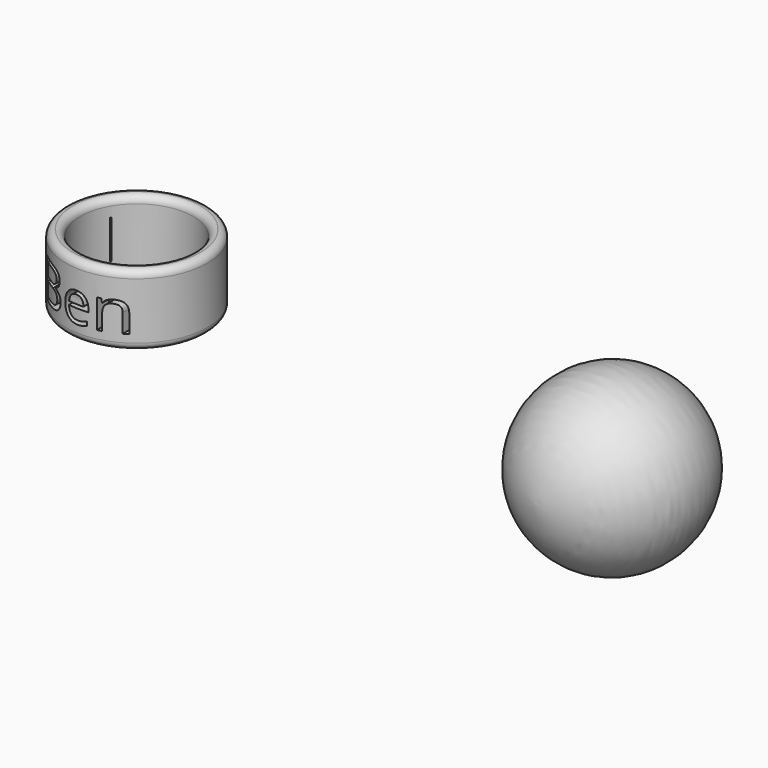
from build123d import *

# Parameters (mm, degrees)
F0_R         = 12.7
F0_R_2       = 10.1142841189
F1_DEPTH     = 12.7
F2_R         = 1.27
F3_TEXT_SIZE = 9.663044087
F4_DEPTH     = 25.4


# Not quite as in the source:
# - Text() gives the source's letters only with a copy of the font that has no kerning and outlines rounded to 1/6400 em; it was checked with that copy


with BuildPart() as f1:
    # F0 (on Top) → F1 (new body)
    with BuildSketch(Plane.XY):
        with Locations((-45.8856523037, 20.2095657587)):
            Circle(F0_R)
        with Locations((-45.8856523037, 20.2095657587)):
            Circle(F0_R_2, mode=Mode.SUBTRACT)
    extrude(amount=F1_DEPTH)

    # F2
    f2_edges = [f1.edges().sort_by_distance(p)[0] for p in [
        (-55.999936, 20.209566, 12.7),
        (-58.585652, 20.209566, 12.7),
        (-58.585652, 20.209566, 0),
        (-55.999936, 20.209566, 0),
    ]]
    fillet(f2_edges, radius=F2_R)

    # F3 (on Front) → F4 (cut)
    with BuildSketch(Plane.XZ):
        with Locations((-55.6278526783, 2.6955050416)):
            Text('Ben', F3_TEXT_SIZE, font='Open Sans', text_align=(TextAlign.LEFT, TextAlign.BOTTOM))
    extrude(amount=-F4_DEPTH, mode=Mode.SUBTRACT)


with BuildPart() as f6:
    # F5 (on Top) → F6 (revolve)
    with BuildSketch(Plane.XY):
        with BuildLine():
            Line((34.9526107311, 8.61391332), (37.6030430198, 39.7565215826))
            ThreePointArc((37.6030430198, 39.7565215826), (21.0088486153, 25.4847037581), (34.9526107311, 8.61391332))
        make_face()
    revolve(axis=Axis((36.2778268754, 24.1852174513, 0), (-0.0847997524, -0.9963980138, 0)))


solid = Compound([f1.part, f6.part])
